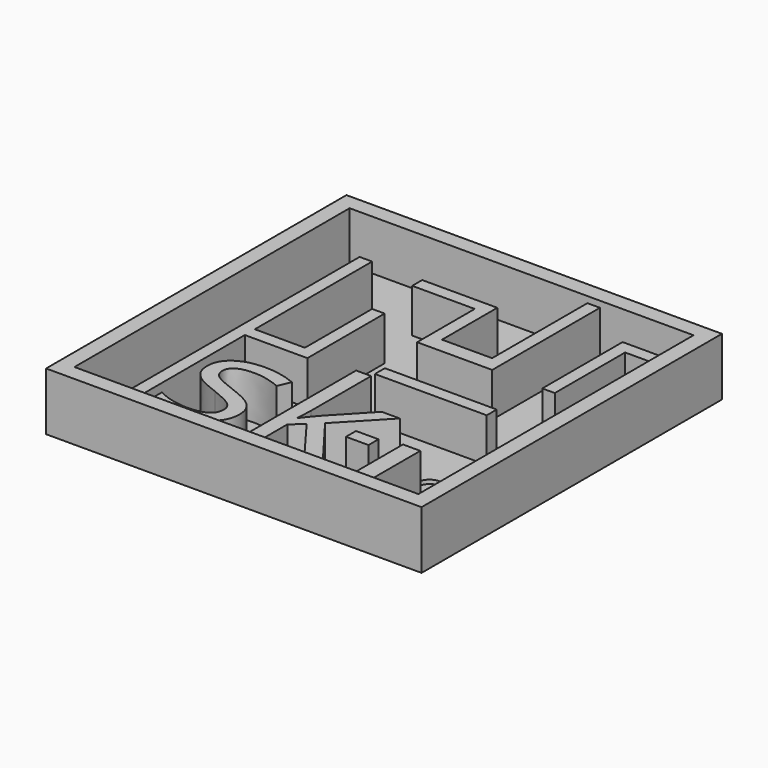
from build123d import *

# Parameters (mm, degrees)
F0_W         = 38.1
F0_H         = 38.1
F1_DEPTH     = 0.79375
F2_W         = 38.1
F2_H         = 38.1
F2_W_2       = 34.8996
F2_H_2       = 34.8996
F3_DEPTH     = 5.08
F4_W         = 11.3512343318
F4_H         = 1.27
F4_W_2       = 2.2840639576
F4_W_3       = 1.756593585
F4_H_2       = 6.8352676787
F4_TEXT_SIZE = 18.9868546631
F5_DEPTH     = 4.445
F6_R         = 1.27
F7_DEPTH     = 0.396875
F8_R         = 1.27
F9_DEPTH     = 0.396875


# Not quite as in the source:
# - Text() gives the source's letters only with a copy of the font that has no kerning and outlines rounded to 1/6400 em; it was checked with that copy


with BuildPart() as f1:
    # F0 (on Top) → F1 (new body)
    with BuildSketch(Plane.XY):
        with Locations((0.4230346531, -1.5346966584)):
            Rectangle(F0_W, F0_H)
    extrude(amount=F1_DEPTH)

    # F2 (on face) → F3 (join)
    with BuildSketch(Plane.XY.offset(0.79375)):
        with Locations((0.4230346531, -1.5346966584)):
            Rectangle(F2_W, F2_H)
        with Locations((0.4230346531, -1.5346966584)):
            Rectangle(F2_W_2, F2_H_2, mode=Mode.SUBTRACT)
    extrude(amount=F3_DEPTH)

    # F4 (on face) → F5 (join)
    with BuildSketch(Plane.XY.offset(0.79375)):
        Polygon((-11.9467653469, 10.8351033416), (-11.9467653469, -18.9844966584), (-10.6767653469, -18.9844966584), (-10.6767653469, -5.313961301), (-4.3267653469, -5.313961301), (-4.3267653469, -4.043961301), (-4.3267653469, 4.4851033416), (-5.5967653469, 4.4851033416), (-5.5967653469, -4.043961301), (-10.6767653469, -4.043961301), (-10.6767653469, 10.8351033416), align=None)
        Polygon((2.0232346531, 10.8351033416), (-5.5967653469, 10.8351033416), (-5.5967653469, 9.5651033416), (0.7532346531, 9.5651033416), (0.7532346531, 7.4549353528), (2.0232346531, 7.4549353528), align=None)
        Polygon((2.0232346531, 3.8244256284), (2.0232346531, 7.4549353528), (0.7532346531, 7.4549353528), (0.7532346531, 2.2536993492), (8.3732346531, 2.2536993492), (8.3732346531, 15.9151033416), (7.1032346531, 15.9151033416), (7.1032346531, 3.8244256284), align=None)
        with Locations((7.2209842298, -3.4613006508)):
            Rectangle(F4_W, F4_H)
        Polygon((13.4532346531, 2.2536993492), (14.7232346531, 2.2536993492), (14.7232346531, 11.1723626032), (17.8728346531, 11.1723626032), (17.8728346531, 12.4423626032), (13.4532346531, 12.4423626032), align=None)
        with Locations((7.6291854493, -13.3042847195)):
            Rectangle(F4_W_2, F4_H)
        with Locations((11.7181604728, -15.5668628191)):
            Rectangle(F4_W_3, F4_H_2)
        with Locations((-10.6767653469, -18.9844966584)):
            Text('sk', F4_TEXT_SIZE, font='Open Sans', text_align=(TextAlign.LEFT, TextAlign.BOTTOM))
    extrude(amount=F5_DEPTH)

    # F6 (on face) → F7 (cut)
    with BuildSketch(Plane.XY.offset(0.79375)):
        with Locations((11.7181604728, -9.8626315594)):
            Circle(F6_R)
    extrude(amount=-F7_DEPTH, mode=Mode.SUBTRACT)

    # F8 (on face) → F9 (cut)
    with BuildSketch(Plane.XY.offset(0.79375)):
        with Locations((-14.4867653469, -15.9693304449)):
            Circle(F8_R)
    extrude(amount=-F9_DEPTH, mode=Mode.SUBTRACT)


solid = f1.part
